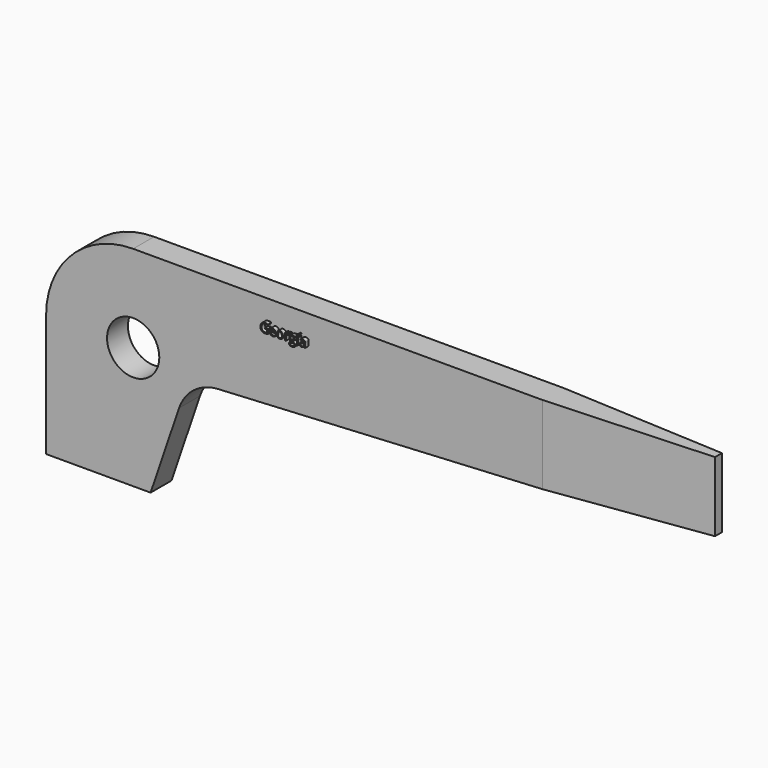
from build123d import *

# Parameters (mm, degrees)
F1_DEPTH     = 2.38125
F2_R         = 2.38125
F3_DEPTH     = 25.4
F5_DEPTH     = 25.4
F6_TEXT_SIZE = 1.1556109207
F7_DEPTH     = 0.396875


# Not quite as in the source:
# - a length typed as a fraction of an inch, garbled in the dataset ("3 / 203.2 mm" for 3/8 in), is restored
# - Text() gives the source's letters only with a copy of the font that has no kerning and outlines rounded to 1/6400 em; it was checked with that copy


with BuildPart() as f1:
    # F0 (on Front) → F1 (new body)
    with BuildSketch(Plane.XZ):
        with BuildLine():
            Line((60.325, 19.05), (7.9375, 19.05))
            ThreePointArc((7.9375, 19.05), (2.3248399243, 16.7251600757), (0, 11.1125))
            Line((0, 11.1125), (0, 0))
            Line((0, 0), (9.525, 0))
            Line((9.525, 0), (12.1173647876, 7.6271664624))
            ThreePointArc((12.1173647876, 7.6271664624), (13.4786145605, 9.5135918491), (15.6631963617, 10.3130942181))
            Line((15.6631963617, 10.3130942181), (60.325, 12.7))
            Line((60.325, 12.7), (60.325, 19.05))
        make_face()
    extrude(amount=F1_DEPTH)

    # F2 (on face) → F3 (cut)
    with BuildSketch(Plane.XZ.offset(2.38125)):
        with Locations((7.9375, 11.1125)):
            Circle(F2_R)
    extrude(amount=-F3_DEPTH, mode=Mode.SUBTRACT)

    # F4 (on face) → F5 (cut)
    with BuildSketch(Plane.XY.offset(19.05)):
        Polygon((60.325, -2.38125), (60.325, -1.5875), (45.24375, -2.38125), align=None)
        Polygon((60.325, 0), (45.24375, 0), (60.325, -0.79375), align=None)
    extrude(amount=-F5_DEPTH, mode=Mode.SUBTRACT)

    # F6 (on face) → F7 (join)
    with BuildSketch(Plane.XZ.offset(2.38125)):
        with Locations((19.7842344642, 16.4441466331)):
            Text('Georgia', F6_TEXT_SIZE, font='Open Sans', text_align=(TextAlign.LEFT, TextAlign.BOTTOM))
    extrude(amount=F7_DEPTH)


solid = f1.part
